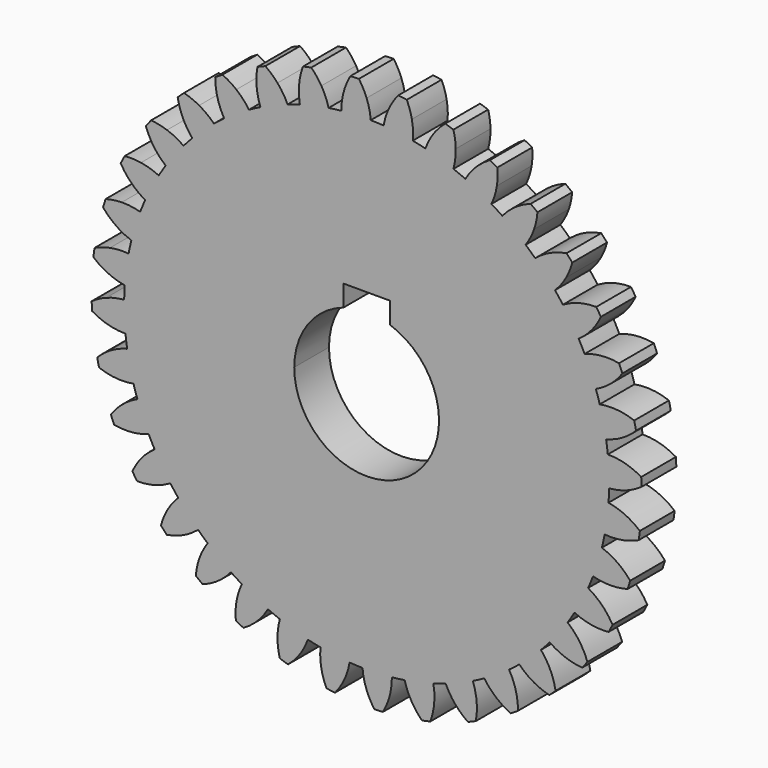
from build123d import *

# Parameters (mm, degrees)
F1_DEPTH = 15
F2_COUNT = 36
F5_DEPTH = 25.4


with BuildPart() as f1:
    # F0 (on Front) → F1 (new body)
    with BuildSketch(Plane.XZ):
        with BuildLine():
            ThreePointArc((-8.7190556623, 83.2949012146), (-56.0528393049, -62.2265353837), (83.75, 0))
            ThreePointArc((83.75, 0), (59.7223189997, 58.7137727735), (1.4262480407, 83.7378547404))
            ThreePointArc((1.4262480407, 83.7378547404), (-3.6531236918, 83.6702885575), (-8.7190556623, 83.2949012146))
        make_face()
        with BuildLine():
            ThreePointArc((-8.7190556623, 83.2949012146), (-3.6531236918, 83.6702885575), (1.4262480407, 83.7378547404))
            ThreePointArc((1.4262480407, 83.7378547404), (0.9377107983, 86.9200786033), (0, 90))
            ThreePointArc((0, 90), (-1.1760420962, 92.5650071018), (-2.663884374, 94.9626438135))
            ThreePointArc((-2.663884374, 94.9626438135), (-4.1438417997, 94.9095810503), (-5.6227922652, 94.833455105))
            ThreePointArc((-5.6227922652, 94.833455105), (-6.8960050455, 92.3152681261), (-7.8440168473, 89.6575228283))
            ThreePointArc((-7.8440168473, 89.6575228283), (-8.509726536, 86.5075945813), (-8.7190556623, 83.2949012146))
        make_face()
    extrude(amount=F1_DEPTH)


with BuildPart() as f2_1:
    # F2: instance of F1
    add(f1.part.rotate(Axis((0, 0, 0), (0, 1, 0)), 1 * 360 / F2_COUNT))


with BuildPart() as f2_2:
    # F2: instance of F1
    add(f1.part.rotate(Axis((0, 0, 0), (0, 1, 0)), 2 * 360 / F2_COUNT))


with BuildPart() as f2_3:
    # F2: instance of F1
    add(f1.part.rotate(Axis((0, 0, 0), (0, 1, 0)), 3 * 360 / F2_COUNT))


with BuildPart() as f2_4:
    # F2: instance of F1
    add(f1.part.rotate(Axis((0, 0, 0), (0, 1, 0)), 4 * 360 / F2_COUNT))


with BuildPart() as f2_5:
    # F2: instance of F1
    add(f1.part.rotate(Axis((0, 0, 0), (0, 1, 0)), 5 * 360 / F2_COUNT))


with BuildPart() as f2_6:
    # F2: instance of F1
    add(f1.part.rotate(Axis((0, 0, 0), (0, 1, 0)), 6 * 360 / F2_COUNT))


with BuildPart() as f2_7:
    # F2: instance of F1
    add(f1.part.rotate(Axis((0, 0, 0), (0, 1, 0)), 7 * 360 / F2_COUNT))


with BuildPart() as f2_8:
    # F2: instance of F1
    add(f1.part.rotate(Axis((0, 0, 0), (0, 1, 0)), 8 * 360 / F2_COUNT))


with BuildPart() as f2_9:
    # F2: instance of F1
    add(f1.part.rotate(Axis((0, 0, 0), (0, 1, 0)), 9 * 360 / F2_COUNT))


with BuildPart() as f2_10:
    # F2: instance of F1
    add(f1.part.rotate(Axis((0, 0, 0), (0, 1, 0)), 10 * 360 / F2_COUNT))


with BuildPart() as f2_11:
    # F2: instance of F1
    add(f1.part.rotate(Axis((0, 0, 0), (0, 1, 0)), 11 * 360 / F2_COUNT))


with BuildPart() as f2_12:
    # F2: instance of F1
    add(f1.part.rotate(Axis((0, 0, 0), (0, 1, 0)), 12 * 360 / F2_COUNT))


with BuildPart() as f2_13:
    # F2: instance of F1
    add(f1.part.rotate(Axis((0, 0, 0), (0, 1, 0)), 13 * 360 / F2_COUNT))


with BuildPart() as f2_14:
    # F2: instance of F1
    add(f1.part.rotate(Axis((0, 0, 0), (0, 1, 0)), 14 * 360 / F2_COUNT))


with BuildPart() as f2_15:
    # F2: instance of F1
    add(f1.part.rotate(Axis((0, 0, 0), (0, 1, 0)), 15 * 360 / F2_COUNT))


with BuildPart() as f2_16:
    # F2: instance of F1
    add(f1.part.rotate(Axis((0, 0, 0), (0, 1, 0)), 16 * 360 / F2_COUNT))


with BuildPart() as f2_17:
    # F2: instance of F1
    add(f1.part.rotate(Axis((0, 0, 0), (0, 1, 0)), 17 * 360 / F2_COUNT))


with BuildPart() as f2_18:
    # F2: instance of F1
    add(f1.part.rotate(Axis((0, 0, 0), (0, 1, 0)), 18 * 360 / F2_COUNT))


with BuildPart() as f2_19:
    # F2: instance of F1
    add(f1.part.rotate(Axis((0, 0, 0), (0, 1, 0)), 19 * 360 / F2_COUNT))


with BuildPart() as f2_20:
    # F2: instance of F1
    add(f1.part.rotate(Axis((0, 0, 0), (0, 1, 0)), 20 * 360 / F2_COUNT))


with BuildPart() as f2_21:
    # F2: instance of F1
    add(f1.part.rotate(Axis((0, 0, 0), (0, 1, 0)), 21 * 360 / F2_COUNT))


with BuildPart() as f2_22:
    # F2: instance of F1
    add(f1.part.rotate(Axis((0, 0, 0), (0, 1, 0)), 22 * 360 / F2_COUNT))


with BuildPart() as f2_23:
    # F2: instance of F1
    add(f1.part.rotate(Axis((0, 0, 0), (0, 1, 0)), 23 * 360 / F2_COUNT))


with BuildPart() as f2_24:
    # F2: instance of F1
    add(f1.part.rotate(Axis((0, 0, 0), (0, 1, 0)), 24 * 360 / F2_COUNT))


with BuildPart() as f2_25:
    # F2: instance of F1
    add(f1.part.rotate(Axis((0, 0, 0), (0, 1, 0)), 25 * 360 / F2_COUNT))


with BuildPart() as f2_26:
    # F2: instance of F1
    add(f1.part.rotate(Axis((0, 0, 0), (0, 1, 0)), 26 * 360 / F2_COUNT))


with BuildPart() as f2_27:
    # F2: instance of F1
    add(f1.part.rotate(Axis((0, 0, 0), (0, 1, 0)), 27 * 360 / F2_COUNT))


with BuildPart() as f2_28:
    # F2: instance of F1
    add(f1.part.rotate(Axis((0, 0, 0), (0, 1, 0)), 28 * 360 / F2_COUNT))


with BuildPart() as f2_29:
    # F2: instance of F1
    add(f1.part.rotate(Axis((0, 0, 0), (0, 1, 0)), 29 * 360 / F2_COUNT))


with BuildPart() as f2_30:
    # F2: instance of F1
    add(f1.part.rotate(Axis((0, 0, 0), (0, 1, 0)), 30 * 360 / F2_COUNT))


with BuildPart() as f2_31:
    # F2: instance of F1
    add(f1.part.rotate(Axis((0, 0, 0), (0, 1, 0)), 31 * 360 / F2_COUNT))


with BuildPart() as f2_32:
    # F2: instance of F1
    add(f1.part.rotate(Axis((0, 0, 0), (0, 1, 0)), 32 * 360 / F2_COUNT))


with BuildPart() as f2_33:
    # F2: instance of F1
    add(f1.part.rotate(Axis((0, 0, 0), (0, 1, 0)), 33 * 360 / F2_COUNT))


with BuildPart() as f2_34:
    # F2: instance of F1
    add(f1.part.rotate(Axis((0, 0, 0), (0, 1, 0)), 34 * 360 / F2_COUNT))


with BuildPart() as f2_35:
    # F2: instance of F1
    add(f1.part.rotate(Axis((0, 0, 0), (0, 1, 0)), 35 * 360 / F2_COUNT))


with BuildPart() as f2_17_1:
    add(f2_17.part)

    # F3: union F2_13, F1, F2_7, F2_18, F2_3, F2_16, F2_8, F2_19, F2_1, F2_34, F2_33, F2_32, F2_31, F2_30, F2_29, F2_28, F2_27, F2_26, F2_25, F2_23, F2_5, F2_2, F2_9, F2_22, F2_24, F2_35, F2_12, F2_10, F2_6, F2_11, F2_14, F2_4, F2_21, F2_20, F2_15
    add(f2_13.part)
    add(f1.part)
    add(f2_7.part)
    add(f2_18.part)
    add(f2_3.part)
    add(f2_16.part)
    add(f2_8.part)
    add(f2_19.part)
    add(f2_1.part)
    add(f2_34.part)
    add(f2_33.part)
    add(f2_32.part)
    add(f2_31.part)
    add(f2_30.part)
    add(f2_29.part)
    add(f2_28.part)
    add(f2_27.part)
    add(f2_26.part)
    add(f2_25.part)
    add(f2_23.part)
    add(f2_5.part)
    add(f2_2.part)
    add(f2_9.part)
    add(f2_22.part)
    add(f2_24.part)
    add(f2_35.part)
    add(f2_12.part)
    add(f2_10.part)
    add(f2_6.part)
    add(f2_11.part)
    add(f2_14.part)
    add(f2_4.part)
    add(f2_21.part)
    add(f2_20.part)
    add(f2_15.part)

    # F4 (on face) → F5 (cut)
    with BuildSketch(Plane(origin=(0, 0, 0), x_dir=(-1, 0, 0), z_dir=(0, 1, 0))):
        with BuildLine():
            ThreePointArc((-8, 23.6854385647), (-14.5773797371, -20.3100960116), (25, 0))
            ThreePointArc((25, 0), (20.3100960116, 14.5773797371), (8, 23.6854385647))
            Line((8, 23.6854385647), (8, 19))
            Line((8, 19), (-8, 19))
            Line((-8, 19), (-8, 23.6854385647))
        make_face()
        with BuildLine():
            Line((8, 19), (8, 23.6854385647))
            ThreePointArc((8, 23.6854385647), (0, 25), (-8, 23.6854385647))
            Line((-8, 23.6854385647), (-8, 19))
            Line((-8, 19), (8, 19))
        make_face()
        with BuildLine():
            ThreePointArc((-8, 23.6854385647), (0, 25), (8, 23.6854385647))
            Line((8, 23.6854385647), (8, 31))
            Line((8, 31), (-8, 31))
            Line((-8, 31), (-8, 23.6854385647))
        make_face()
    extrude(amount=-F5_DEPTH, mode=Mode.SUBTRACT)


solid = f2_17_1.part
